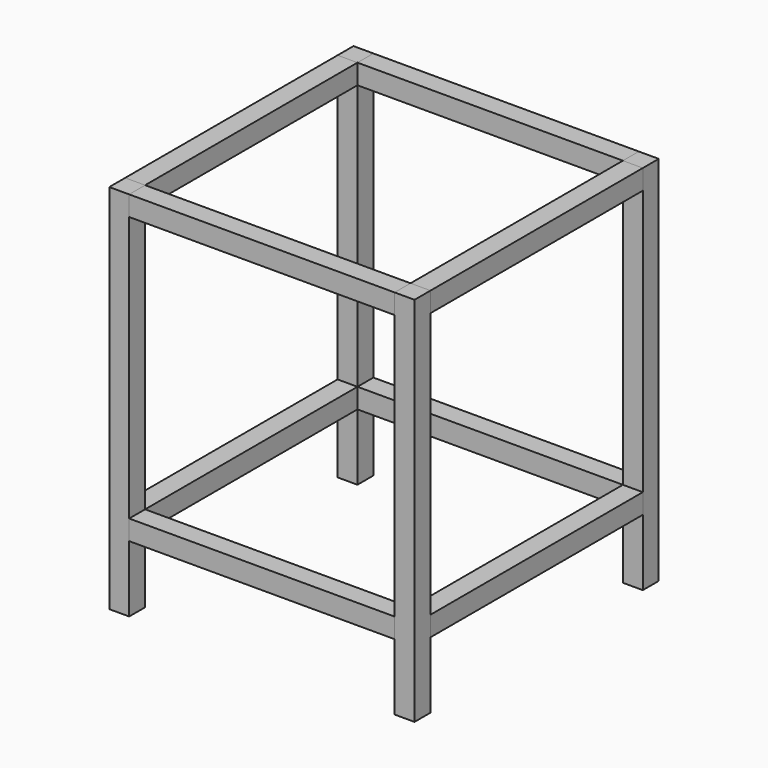
from build123d import *

# Parameters (mm, degrees)
F3_W     = 30
F3_H     = 30
F4_DEPTH = 230
F5_W     = 30
F5_H     = 30
F6_DEPTH = 200
F7_W     = 30
F7_H     = 30
F8_DEPTH = 200
F9_DEPTH = 100


with BuildPart() as f4:
    # F3 (on Top) → F4 (new body, symmetric)
    with BuildSketch(Plane.XY):
        with Locations((-215, 215)):
            Rectangle(F3_W, F3_H)
    extrude(amount=F4_DEPTH, both=True)

    # F9#3 (add): a face of the model
    f9_3_faces = [f4.faces().sort_by_distance(p)[0] for p in [
        (-215, 215, -230),
    ]]
    extrude(f9_3_faces, amount=F9_DEPTH)


with BuildPart() as f4b:
    # F3 (on Top) → F4, piece 2 (new body, symmetric)
    with BuildSketch(Plane.XY):
        with Locations((215, 215)):
            Rectangle(F3_W, F3_H)
    extrude(amount=F4_DEPTH, both=True)

    # F9#4 (add): a face of the model
    f9_4_faces = [f4b.faces().sort_by_distance(p)[0] for p in [
        (215, 215, -230),
    ]]
    extrude(f9_4_faces, amount=F9_DEPTH)


with BuildPart() as f4c:
    # F3 (on Top) → F4, piece 3 (new body, symmetric)
    with BuildSketch(Plane.XY):
        with Locations((215, -215)):
            Rectangle(F3_W, F3_H)
    extrude(amount=F4_DEPTH, both=True)

    # F9#2 (add): a face of the model
    f9_2_faces = [f4c.faces().sort_by_distance(p)[0] for p in [
        (215, -215, -230),
    ]]
    extrude(f9_2_faces, amount=F9_DEPTH)


with BuildPart() as f4d:
    # F3 (on Top) → F4, piece 4 (new body, symmetric)
    with BuildSketch(Plane.XY):
        with Locations((-215, -215)):
            Rectangle(F3_W, F3_H)
    extrude(amount=F4_DEPTH, both=True)

    # F9 (add): a face of the model
    f9_faces = [f4d.faces().sort_by_distance(p)[0] for p in [
        (-215, -215, -230),
    ]]
    extrude(f9_faces, amount=F9_DEPTH)


with BuildPart() as f6:
    # F5 (on Front) → F6 (new body, symmetric)
    with BuildSketch(Plane.XZ):
        with Locations((-215, 215)):
            Rectangle(F5_W, F5_H)
    extrude(amount=F6_DEPTH, both=True)


with BuildPart() as f6b:
    # F5 (on Front) → F6, piece 2 (new body, symmetric)
    with BuildSketch(Plane.XZ):
        with Locations((215, 215)):
            Rectangle(F5_W, F5_H)
    extrude(amount=F6_DEPTH, both=True)


with BuildPart() as f6c:
    # F5 (on Front) → F6, piece 3 (new body, symmetric)
    with BuildSketch(Plane.XZ):
        with Locations((-215, -215)):
            Rectangle(F5_W, F5_H)
    extrude(amount=F6_DEPTH, both=True)


with BuildPart() as f6d:
    # F5 (on Front) → F6, piece 4 (new body, symmetric)
    with BuildSketch(Plane.XZ):
        with Locations((215, -215)):
            Rectangle(F5_W, F5_H)
    extrude(amount=F6_DEPTH, both=True)


with BuildPart() as f8:
    # F7 (on Right) → F8 (new body, symmetric)
    with BuildSketch(Plane.YZ):
        with Locations((-215, 215)):
            Rectangle(F7_W, F7_H)
    extrude(amount=F8_DEPTH, both=True)


with BuildPart() as f8b:
    # F7 (on Right) → F8, piece 2 (new body, symmetric)
    with BuildSketch(Plane.YZ):
        with Locations((215, 215)):
            Rectangle(F7_W, F7_H)
    extrude(amount=F8_DEPTH, both=True)


with BuildPart() as f8c:
    # F7 (on Right) → F8, piece 3 (new body, symmetric)
    with BuildSketch(Plane.YZ):
        with Locations((215, -215)):
            Rectangle(F7_W, F7_H)
    extrude(amount=F8_DEPTH, both=True)


with BuildPart() as f8d:
    # F7 (on Right) → F8, piece 4 (new body, symmetric)
    with BuildSketch(Plane.YZ):
        with Locations((-215, -215)):
            Rectangle(F7_W, F7_H)
    extrude(amount=F8_DEPTH, both=True)


solid = Compound([f4.part, f4b.part, f4c.part, f4d.part, f6.part, f6b.part, f6c.part, f6d.part, f8.part, f8b.part, f8c.part, f8d.part])
